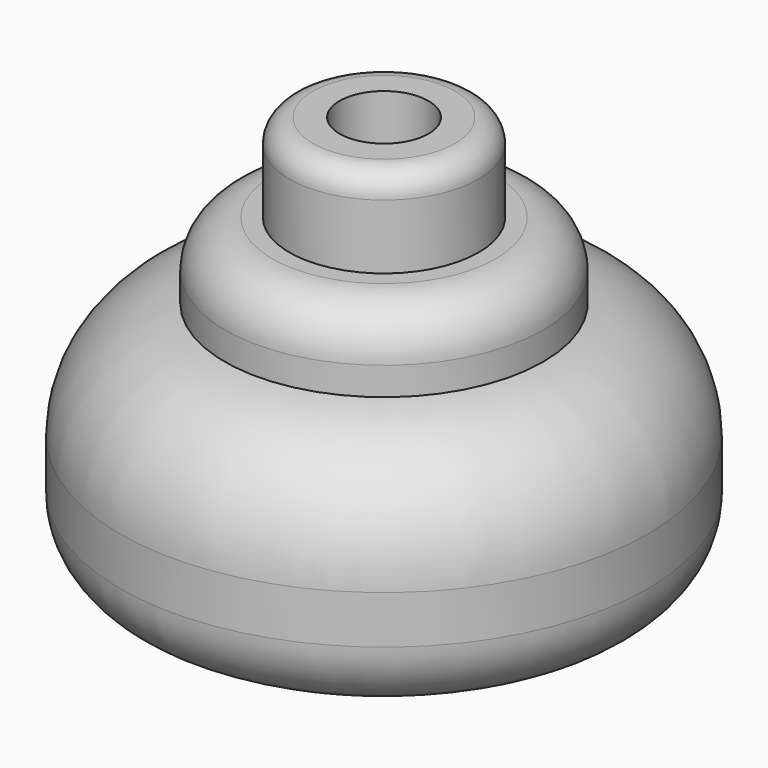
from build123d import *

# Parameters (mm, degrees)
F2_R     = 5.08
F4_R     = 7.62
F5_R     = 2.54
F6_R     = 4.7752
F7_DEPTH = 11.43
F8_R     = 1.6002
F9_DEPTH = 19.685


# Not quite as in the source:
# - a fillet or chamfer that OpenCascade refuses, or shapes differently, is made with other operations: its cross-section is extruded or revolved along the edge and cut away or added


with BuildPart() as f1:
    # F0 (on Front) → F1 (revolve)
    with BuildSketch(Plane.XZ):
        Polygon((0, 48.26), (0, 0), (5.4729898483, 5.3019602149), (28.3329898483, 5.3019602149), (28.3329898483, 30.7019602149), (17.0898887448, 30.7019602149), (17.0898887448, 38.7901112552), (10.16, 38.7901112552), (10.16, 48.26), align=None)
    revolve(axis=Axis((0, 0, 24.13), (0, 0, -1)))

    # F2
    f2_edges = [f1.edges().sort_by_distance(p)[0] for p in [
        (-17.089889, 0, 38.790111),
    ]]
    fillet(f2_edges, radius=F2_R)

    # F3: fillet of radius 12.7 on 1 edges, made by hand

    # F3_s1 → F3_t2 (revolve, cut)
    with BuildSketch(Plane.XZ):
        with BuildLine():
            ThreePointArc((17.0898887448, 30.7019602149), (25.1143562052, 26.5352808999), (28.3329898483, 18.085802099))
            Line((28.3329898483, 18.085802099), (28.3329898483, 30.7019602149))
            Line((28.3329898483, 30.7019602149), (17.0898887448, 30.7019602149))
        make_face()
    revolve(axis=Axis((0, 0, 30.7019602149), (0, 0, -1)), mode=Mode.SUBTRACT)

    # F4
    f4_edges = [f1.edges().sort_by_distance(p)[0] for p in [
        (-28.33299, 0, 5.30196),
    ]]
    fillet(f4_edges, radius=F4_R)

    # F5
    f5_edges = [f1.edges().sort_by_distance(p)[0] for p in [
        (-10.16, 0, 48.26),
    ]]
    fillet(f5_edges, radius=F5_R)

    # F6 (on face) → F7 (cut)
    with BuildSketch(Plane.XY.offset(48.26)):
        Circle(F6_R)
    extrude(amount=-F7_DEPTH, mode=Mode.SUBTRACT)

    # F8 (on Top) → F9 (cut)
    with BuildSketch(Plane.XY):
        Circle(F8_R)
    extrude(amount=F9_DEPTH, mode=Mode.SUBTRACT)


solid = f1.part
